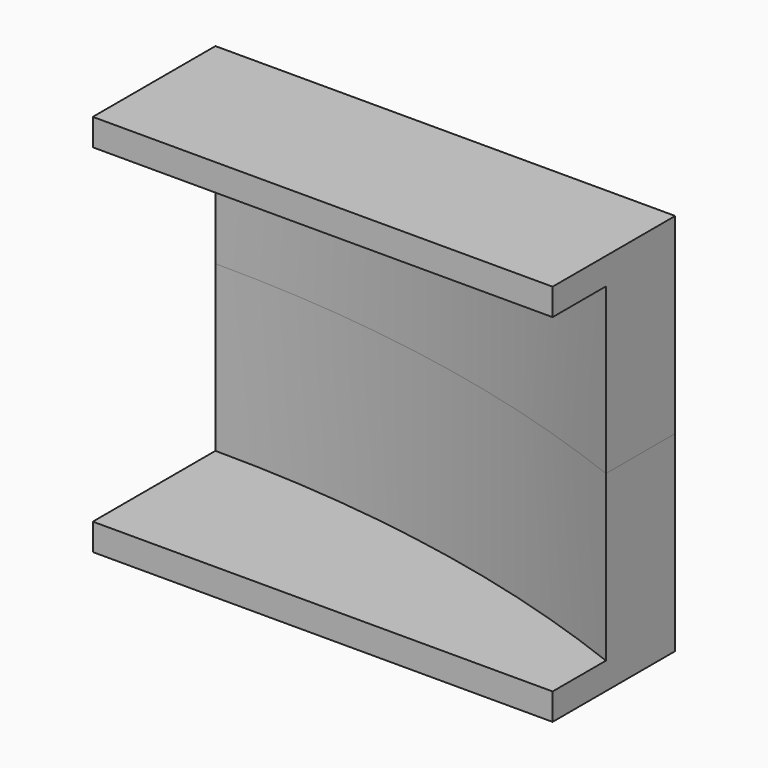
from build123d import *

# Parameters (mm, degrees)
F1_W     = 30
F1_H     = 10
F2_DEPTH = 12.5
F4_DEPTH = 10.75


# Not quite as in the source:
# - a feature names something its author has since deleted; it is built from what else it names


with BuildPart() as f2:
    # F1 (on Top) → F2 (new body)
    with BuildSketch(Plane.XY):
        with Locations((15, -5)):
            Rectangle(F1_W, F1_H)
    extrude(amount=F2_DEPTH)

    # F3 (on face) → F4 (cut)
    with BuildSketch(Plane.XY.offset(12.5)):
        with BuildLine():
            Line((30, -10), (30, -5.6478692553))
            ThreePointArc((30, -5.6478692553), (15.2635057173, -1.4242613773), (0, 0))
            Line((0, 0), (0, -10))
            Line((0, -10), (30, -10))
        make_face()
    extrude(amount=-F4_DEPTH, mode=Mode.SUBTRACT)


with BuildPart() as f5_1:
    # F5: instance of F2
    add(f2.part.mirror(Plane(origin=(22.5523055591, -1.6839325629, 12.5), x_dir=(1, 0, 0), z_dir=(0, 0, 1))))


solid = Compound([f2.part, f5_1.part])
